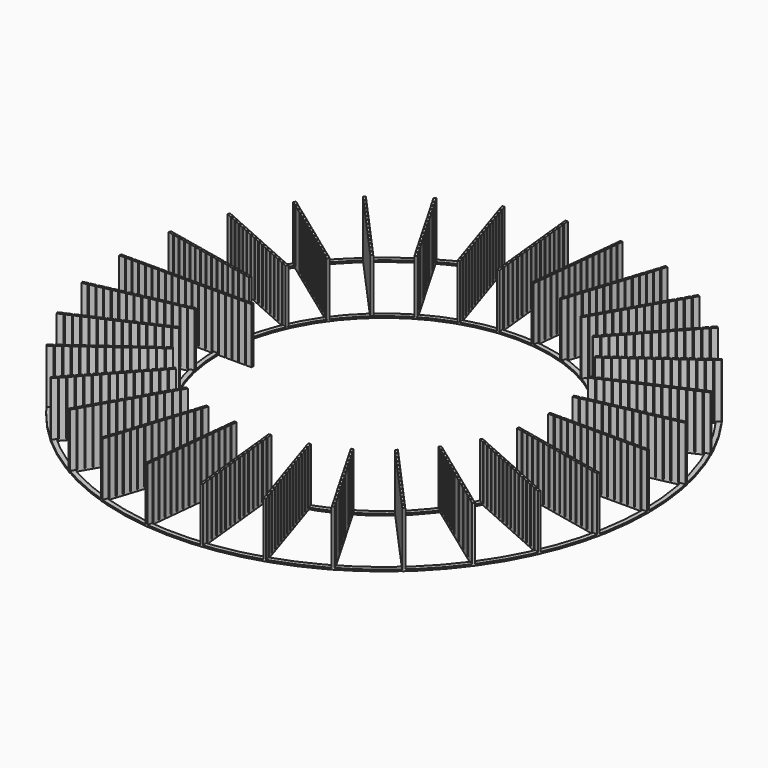
from build123d import *

# Parameters (mm, degrees)
F0_W     = 17.5
F0_H     = 0.42
F1_DEPTH = 0.3
F2_W     = 1
F2_H     = 0.42
F3_DEPTH = 10
F5_COUNT = 30
F6_R     = 47.5
F6_R_2   = 46.7
F7_DEPTH = 0.3
F8_R     = 30.5
F8_R_2   = 29.7
F9_DEPTH = 0.3


with BuildPart() as f1:
    # F0 (on Top) → F1 (new body)
    with BuildSketch(Plane.XY):
        with Locations((-38.75, 0)):
            Rectangle(F0_W, F0_H)
    extrude(amount=F1_DEPTH)

    # F2 (on Top) → F3 (join)
    with BuildSketch(Plane.XY):
        with Locations((-47, 0)):
            Rectangle(F2_W, F2_H)
        with Locations((-45.8, 0)):
            Rectangle(F2_W, F2_H)
        with Locations((-44.6, 0)):
            Rectangle(F2_W, F2_H)
        with Locations((-43.4, 0)):
            Rectangle(F2_W, F2_H)
        with Locations((-42.2, 0)):
            Rectangle(F2_W, F2_H)
        with Locations((-41, 0)):
            Rectangle(F2_W, F2_H)
        with Locations((-39.8, 0)):
            Rectangle(F2_W, F2_H)
        with Locations((-38.6, 0)):
            Rectangle(F2_W, F2_H)
        with Locations((-37.4, 0)):
            Rectangle(F2_W, F2_H)
        with Locations((-36.2, 0)):
            Rectangle(F2_W, F2_H)
        with Locations((-35, 0)):
            Rectangle(F2_W, F2_H)
        with Locations((-33.8, 0)):
            Rectangle(F2_W, F2_H)
        with Locations((-32.6, 0)):
            Rectangle(F2_W, F2_H)
        with Locations((-31.4, 0)):
            Rectangle(F2_W, F2_H)
        with Locations((-30.2, 0)):
            Rectangle(F2_W, F2_H)
    extrude(amount=F3_DEPTH)


with BuildPart() as f3:
    # F2 (on Top) → F3, piece 2 (new body)
    with BuildSketch(Plane.XY):
        with Locations((-29, 0)):
            Rectangle(F2_W, F2_H)
    extrude(amount=F3_DEPTH)


with BuildPart() as f3b:
    # F2 (on Top) → F3, piece 3 (new body)
    with BuildSketch(Plane.XY):
        with Locations((-27.8, 0)):
            Rectangle(F2_W, F2_H)
    extrude(amount=F3_DEPTH)


with BuildPart() as f3c:
    # F2 (on Top) → F3, piece 4 (new body)
    with BuildSketch(Plane.XY):
        with Locations((-26.6, 0)):
            Rectangle(F2_W, F2_H)
    extrude(amount=F3_DEPTH)


with BuildPart() as f3d:
    # F2 (on Top) → F3, piece 5 (new body)
    with BuildSketch(Plane.XY):
        with Locations((-25.4, 0)):
            Rectangle(F2_W, F2_H)
    extrude(amount=F3_DEPTH)


with BuildPart() as f3e:
    # F2 (on Top) → F3, piece 6 (new body)
    with BuildSketch(Plane.XY):
        with Locations((-24.2, 0)):
            Rectangle(F2_W, F2_H)
    extrude(amount=F3_DEPTH)


with BuildPart() as f5_1:
    # F5: instance of F1
    add(f1.part.rotate(Axis((0, 0, 10.7473339885), (0, 0, 1)), 1 * 360 / F5_COUNT))


with BuildPart() as f5_2:
    # F5: instance of F1
    add(f1.part.rotate(Axis((0, 0, 10.7473339885), (0, 0, 1)), 2 * 360 / F5_COUNT))


with BuildPart() as f5_3:
    # F5: instance of F1
    add(f1.part.rotate(Axis((0, 0, 10.7473339885), (0, 0, 1)), 3 * 360 / F5_COUNT))


with BuildPart() as f5_4:
    # F5: instance of F1
    add(f1.part.rotate(Axis((0, 0, 10.7473339885), (0, 0, 1)), 4 * 360 / F5_COUNT))


with BuildPart() as f5_5:
    # F5: instance of F1
    add(f1.part.rotate(Axis((0, 0, 10.7473339885), (0, 0, 1)), 5 * 360 / F5_COUNT))


with BuildPart() as f5_6:
    # F5: instance of F1
    add(f1.part.rotate(Axis((0, 0, 10.7473339885), (0, 0, 1)), 6 * 360 / F5_COUNT))


with BuildPart() as f5_7:
    # F5: instance of F1
    add(f1.part.rotate(Axis((0, 0, 10.7473339885), (0, 0, 1)), 7 * 360 / F5_COUNT))


with BuildPart() as f5_8:
    # F5: instance of F1
    add(f1.part.rotate(Axis((0, 0, 10.7473339885), (0, 0, 1)), 8 * 360 / F5_COUNT))


with BuildPart() as f5_9:
    # F5: instance of F1
    add(f1.part.rotate(Axis((0, 0, 10.7473339885), (0, 0, 1)), 9 * 360 / F5_COUNT))


with BuildPart() as f5_10:
    # F5: instance of F1
    add(f1.part.rotate(Axis((0, 0, 10.7473339885), (0, 0, 1)), 10 * 360 / F5_COUNT))


with BuildPart() as f5_11:
    # F5: instance of F1
    add(f1.part.rotate(Axis((0, 0, 10.7473339885), (0, 0, 1)), 11 * 360 / F5_COUNT))


with BuildPart() as f5_12:
    # F5: instance of F1
    add(f1.part.rotate(Axis((0, 0, 10.7473339885), (0, 0, 1)), 12 * 360 / F5_COUNT))


with BuildPart() as f5_13:
    # F5: instance of F1
    add(f1.part.rotate(Axis((0, 0, 10.7473339885), (0, 0, 1)), 13 * 360 / F5_COUNT))


with BuildPart() as f5_14:
    # F5: instance of F1
    add(f1.part.rotate(Axis((0, 0, 10.7473339885), (0, 0, 1)), 14 * 360 / F5_COUNT))


with BuildPart() as f5_15:
    # F5: instance of F1
    add(f1.part.rotate(Axis((0, 0, 10.7473339885), (0, 0, 1)), 15 * 360 / F5_COUNT))


with BuildPart() as f5_16:
    # F5: instance of F1
    add(f1.part.rotate(Axis((0, 0, 10.7473339885), (0, 0, 1)), 16 * 360 / F5_COUNT))


with BuildPart() as f5_17:
    # F5: instance of F1
    add(f1.part.rotate(Axis((0, 0, 10.7473339885), (0, 0, 1)), 17 * 360 / F5_COUNT))


with BuildPart() as f5_18:
    # F5: instance of F1
    add(f1.part.rotate(Axis((0, 0, 10.7473339885), (0, 0, 1)), 18 * 360 / F5_COUNT))


with BuildPart() as f5_19:
    # F5: instance of F1
    add(f1.part.rotate(Axis((0, 0, 10.7473339885), (0, 0, 1)), 19 * 360 / F5_COUNT))


with BuildPart() as f5_20:
    # F5: instance of F1
    add(f1.part.rotate(Axis((0, 0, 10.7473339885), (0, 0, 1)), 20 * 360 / F5_COUNT))


with BuildPart() as f5_21:
    # F5: instance of F1
    add(f1.part.rotate(Axis((0, 0, 10.7473339885), (0, 0, 1)), 21 * 360 / F5_COUNT))


with BuildPart() as f5_22:
    # F5: instance of F1
    add(f1.part.rotate(Axis((0, 0, 10.7473339885), (0, 0, 1)), 22 * 360 / F5_COUNT))


with BuildPart() as f5_23:
    # F5: instance of F1
    add(f1.part.rotate(Axis((0, 0, 10.7473339885), (0, 0, 1)), 23 * 360 / F5_COUNT))


with BuildPart() as f5_24:
    # F5: instance of F1
    add(f1.part.rotate(Axis((0, 0, 10.7473339885), (0, 0, 1)), 24 * 360 / F5_COUNT))


with BuildPart() as f5_25:
    # F5: instance of F1
    add(f1.part.rotate(Axis((0, 0, 10.7473339885), (0, 0, 1)), 25 * 360 / F5_COUNT))


with BuildPart() as f5_26:
    # F5: instance of F1
    add(f1.part.rotate(Axis((0, 0, 10.7473339885), (0, 0, 1)), 26 * 360 / F5_COUNT))


with BuildPart() as f5_27:
    # F5: instance of F1
    add(f1.part.rotate(Axis((0, 0, 10.7473339885), (0, 0, 1)), 27 * 360 / F5_COUNT))


with BuildPart() as f5_28:
    # F5: instance of F1
    add(f1.part.rotate(Axis((0, 0, 10.7473339885), (0, 0, 1)), 28 * 360 / F5_COUNT))


with BuildPart() as f5_29:
    # F5: instance of F1
    add(f1.part.rotate(Axis((0, 0, 10.7473339885), (0, 0, 1)), 29 * 360 / F5_COUNT))


with BuildPart() as f7:
    # F6 (on face) → F7 (new body)
    with BuildSketch(Plane(origin=(0, 0, 0), x_dir=(1, 0, 0), z_dir=(0, 0, -1))):
        Circle(F6_R)
        Circle(F6_R_2, mode=Mode.SUBTRACT)
    extrude(amount=-F7_DEPTH)


with BuildPart() as f9:
    # F8 (on face) → F9 (new body)
    with BuildSketch(Plane(origin=(0, 0, 0), x_dir=(1, 0, 0), z_dir=(0, 0, -1))):
        Circle(F8_R)
        Circle(F8_R_2, mode=Mode.SUBTRACT)
    extrude(amount=-F9_DEPTH)


solid = Compound([f1.part, f3.part, f3b.part, f3c.part, f3d.part, f3e.part, f5_1.part, f5_2.part, f5_3.part, f5_4.part, f5_5.part, f5_6.part, f5_7.part, f5_8.part, f5_9.part, f5_10.part, f5_11.part, f5_12.part, f5_13.part, f5_14.part, f5_15.part, f5_16.part, f5_17.part, f5_18.part, f5_19.part, f5_20.part, f5_21.part, f5_22.part, f5_23.part, f5_24.part, f5_25.part, f5_26.part, f5_27.part, f5_28.part, f5_29.part, f7.part, f9.part])
